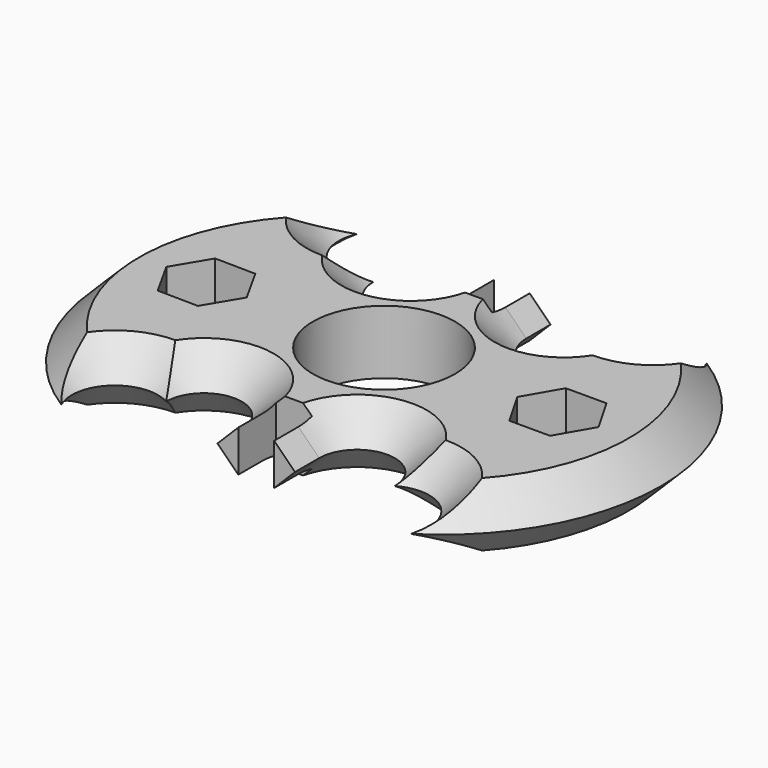
from build123d import *

# Parameters (mm, degrees)
F0_R         = 11.125
F1_DEPTH     = 10
F2_T1_DEPTH  = 17.5952575274
F2_T3_DEPTH  = 17.5952575274
F2_T6_ANGLE  = 359.64
F2_T8_ANGLE  = 359.64
F2_T10_ANGLE = 158.7108465942
F2_T12_ANGLE = 359.64
F2_T14_ANGLE = 359.64
F2_T16_ANGLE = 359.64
F2_T18_ANGLE = 359.64
F2_T20_ANGLE = 158.7108465942
F2_T22_ANGLE = 359.64
F2_T24_ANGLE = 359.64
F2_T26_ANGLE = 359.64
F2_T28_ANGLE = 158.7108465942
F2_T30_ANGLE = 359.64
F2_T32_ANGLE = 359.64
F2_T34_ANGLE = 359.64
F2_T36_ANGLE = 359.64
F2_T38_ANGLE = 359.64
F2_T40_ANGLE = 359.64
F2_T42_ANGLE = 158.7108465942
F2_T44_ANGLE = 359.64


# Not quite as in the source:
# - a fillet or chamfer that OpenCascade refuses, or shapes differently, is made with other operations: its cross-section is extruded or revolved along the edge and cut away or added


with BuildPart() as f1:
    # F0 (on Top) → F1 (new body)
    with BuildSketch(Plane.XY):
        with BuildLine():
            Line((-2.8125022072, -17.6151320338), (0, -17.6151320338))
            Line((0, -17.6151320338), (2.8125022072, -17.6151320338))
            Line((2.8125022072, -17.6151320338), (2.8125022072, -25.0164493918))
            Line((2.8125022072, -25.0164493918), (6.0690809041, -25.0164493918))
            Line((6.0690809041, -25.0164493918), (6.0690809041, -20.2796068043))
            ThreePointArc((6.0690809041, -20.2796068043), (11.9901318103, -14.3585558981), (17.9111827165, -20.2796068043))
            ThreePointArc((17.9111827165, -20.2796068043), (25.8046814323, -21.1516241303), (27.4031855301, -28.930603552))
            ThreePointArc((27.4031855301, -28.930603552), (43.3717109263, 0), (27.4031855301, 28.930603552))
            ThreePointArc((27.4031855301, 28.930603552), (25.8046814323, 21.1516241303), (17.9111827165, 20.2796068043))
            ThreePointArc((17.9111827165, 20.2796068043), (11.9901318103, 14.3585558981), (6.0690809041, 20.2796068043))
            Line((6.0690809041, 20.2796068043), (6.0690809041, 25.0164493918))
            Line((6.0690809041, 25.0164493918), (2.8125022072, 25.0164493918))
            Line((2.8125022072, 25.0164493918), (2.8125022072, 17.6151320338))
            Line((2.8125022072, 17.6151320338), (0, 17.6151320338))
            Line((0, 17.6151320338), (-2.8125022072, 17.6151320338))
            Line((-2.8125022072, 17.6151320338), (-2.8125022072, 25.0164493918))
            Line((-2.8125022072, 25.0164493918), (-6.0690809041, 25.0164493918))
            Line((-6.0690809041, 25.0164493918), (-6.0690809041, 20.2796068043))
            ThreePointArc((-6.0690809041, 20.2796068043), (-11.9901318103, 14.3585558981), (-17.9111827165, 20.2796068043))
            ThreePointArc((-17.9111827165, 20.2796068043), (-25.8046814323, 21.1516241303), (-27.4031855301, 28.930603552))
            ThreePointArc((-27.4031855301, 28.930603552), (-43.3717109263, 0), (-27.4031855301, -28.930603552))
            ThreePointArc((-27.4031855301, -28.930603552), (-25.8046814323, -21.1516241303), (-17.9111827165, -20.2796068043))
            ThreePointArc((-17.9111827165, -20.2796068043), (-11.9901318103, -14.3585558981), (-6.0690809041, -20.2796068043))
            Line((-6.0690809041, -20.2796068043), (-6.0690809041, -25.0164493918))
            Line((-6.0690809041, -25.0164493918), (-2.8125022072, -25.0164493918))
            Line((-2.8125022072, -25.0164493918), (-2.8125022072, -17.6151320338))
        make_face()
        Polygon((-30.9119913686, 5.5693711821), (-24.537748198, 5.4711418492), (-21.4356957103, -0.0982293328), (-24.7078863932, -5.5693711821), (-31.0821295639, -5.4711418492), (-34.1841820515, 0.0982293328), align=None, mode=Mode.SUBTRACT)
        Circle(F0_R, mode=Mode.SUBTRACT)
        Polygon((20.875, 0), (24.0625, 5.5209119491), (30.4375, 5.5209119491), (33.625, 0), (30.4375, -5.5209119491), (24.0625, -5.5209119491), align=None, mode=Mode.SUBTRACT)
    extrude(amount=F1_DEPTH)

    # F2: chamfer of 5 on 20 edges, made by hand

    # F2_s2 → F2_t1 (cut)
    with BuildSketch(Plane.XZ.offset(-37.8748643317)):
        Polygon((-6.0690809041, 5), (-1.0690809041, 0), (-6.0690809041, 0), align=None)
        Polygon((6.0690809041, 5), (1.0690809041, 0), (6.0690809041, 0), align=None)
        Polygon((1.0690809041, 10), (6.0690809041, 5), (6.0690809041, 10), align=None)
        Polygon((-1.0690809041, 10), (-6.0690809041, 5), (-6.0690809041, 10), align=None)
    extrude(amount=F2_T1_DEPTH, mode=Mode.SUBTRACT)

    # F2_s4 → F2_t3 (cut)
    with BuildSketch(Plane.XZ.offset(20.2796068043)):
        Polygon((-1.0690809041, 0), (-6.0690809041, 5), (-6.0690809041, 0), align=None)
        Polygon((6.0690809041, 5), (1.0690809041, 0), (6.0690809041, 0), align=None)
        Polygon((1.0690809041, 10), (6.0690809041, 5), (6.0690809041, 10), align=None)
        Polygon((-1.0690809041, 10), (-6.0690809041, 5), (-6.0690809041, 10), align=None)
    extrude(amount=F2_T3_DEPTH, mode=Mode.SUBTRACT)

    # F2_s5 → F2_t6 (revolve, cut)
    with BuildSketch(Plane(origin=(-24.5672156268, 22.5322183518, 0), x_dir=(0, 0, 1), z_dir=(-0.7369707586, 0.6759246267, 0))):
        Polygon((10, 16.6434047939), (5, 11.6434047939), (10, 11.6434047939), align=None)
    revolve(axis=Axis((-21.2587402157, 26.1394987159, 10), (0, 0, -1)), revolution_arc=F2_T6_ANGLE, mode=Mode.SUBTRACT)

    # F2_s7 → F2_t8 (revolve, cut)
    with BuildSketch(Plane.XZ.offset(-20.2796068043)):
        Polygon((-1.0690809041, 10), (-6.0690809041, 5), (-6.0690809041, 10), align=None)
    revolve(axis=Axis((-11.9901318103, 20.2796068043, 10), (0, 0, -1)), revolution_arc=F2_T8_ANGLE, mode=Mode.SUBTRACT)

    # F2_s9 → F2_t10 (revolve, cut)
    with BuildSketch(Plane(origin=(-8.8670439331, -1.6665634724, 0), x_dir=(0, 0, 1), z_dir=(0.9827919356, 0.1847160286, 0))):
        Polygon((10, -30.8871798498), (5, -35.8871798498), (10, -35.8871798498), align=None)
    revolve(axis=Axis((-9.1802750199, 0, 10), (0, 0, 1)), revolution_arc=F2_T10_ANGLE, mode=Mode.SUBTRACT)

    # F2_s11 → F2_t12 (revolve, cut)
    with BuildSketch(Plane(origin=(-24.6850209159, -22.3563277123, 0), x_dir=(0, 0, 1), z_dir=(0.7412031432, 0.6712807911, 0))):
        Polygon((10, 16.8527592984), (5, 11.8527592984), (10, 11.8527592984), align=None)
    revolve(axis=Axis((-21.2587402157, -26.1394987159, 10), (0, 0, -1)), revolution_arc=F2_T12_ANGLE, mode=Mode.SUBTRACT)

    # F2_s13 → F2_t14 (revolve, cut)
    with BuildSketch(Plane(origin=(-0.1278905192, -20.3541404453, 0), x_dir=(0, 0, 1), z_dir=(0.006283144, 0.9999802609, 0))):
        Polygon((5, -5.9414245401), (10, -0.9414245401), (10, -5.9414245401), align=None)
    revolve(axis=Axis((-11.9901318103, -20.2796068043, 10), (0, 0, -1)), revolution_arc=F2_T14_ANGLE, mode=Mode.SUBTRACT)

    # F2_s15 → F2_t16 (revolve, cut)
    with BuildSketch(Plane.XZ.offset(20.2796068043)):
        Polygon((1.0690809041, 10), (6.0690809041, 5), (6.0690809041, 10), align=None)
    revolve(axis=Axis((11.9901318103, -20.2796068043, 10), (0, 0, -1)), revolution_arc=F2_T16_ANGLE, mode=Mode.SUBTRACT)

    # F2_s17 → F2_t18 (revolve, cut)
    with BuildSketch(Plane(origin=(24.5672156268, -22.5322183518, 0), x_dir=(0, 0, 1), z_dir=(0.7369707586, -0.6759246267, 0))):
        Polygon((10, 16.6434047939), (5, 11.6434047939), (10, 11.6434047939), align=None)
    revolve(axis=Axis((21.2587402157, -26.1394987159, 10), (0, 0, -1)), revolution_arc=F2_T18_ANGLE, mode=Mode.SUBTRACT)

    # F2_s19 → F2_t20 (revolve, cut)
    with BuildSketch(Plane(origin=(8.8670439331, 1.6665634724, 0), x_dir=(0, 0, 1), z_dir=(-0.9827919356, -0.1847160286, 0))):
        Polygon((10, -30.8871798498), (5, -35.8871798498), (10, -35.8871798498), align=None)
    revolve(axis=Axis((9.1802750199, 0, 10), (0, 0, 1)), revolution_arc=F2_T20_ANGLE, mode=Mode.SUBTRACT)

    # F2_s21 → F2_t22 (revolve, cut)
    with BuildSketch(Plane(origin=(24.6850209159, 22.3563277123, 0), x_dir=(0, 0, 1), z_dir=(-0.7412031432, -0.6712807911, 0))):
        Polygon((10, 16.8527592984), (5, 11.8527592984), (10, 11.8527592984), align=None)
    revolve(axis=Axis((21.2587402157, 26.1394987159, 10), (0, 0, -1)), revolution_arc=F2_T22_ANGLE, mode=Mode.SUBTRACT)

    # F2_s23 → F2_t24 (revolve, cut)
    with BuildSketch(Plane(origin=(0.1278905192, 20.3541404453, 0), x_dir=(0, 0, 1), z_dir=(-0.006283144, -0.9999802609, 0))):
        Polygon((10, -0.9414245401), (5, -5.9414245401), (10, -5.9414245401), align=None)
    revolve(axis=Axis((11.9901318103, 20.2796068043, 10), (0, 0, -1)), revolution_arc=F2_T24_ANGLE, mode=Mode.SUBTRACT)

    # F2_s25 → F2_t26 (revolve, cut)
    with BuildSketch(Plane(origin=(24.6850209159, 22.3563277123, 0), x_dir=(0, 0, 1), z_dir=(-0.7412031432, -0.6712807911, 0))):
        Polygon((5, 11.8527592984), (0, 16.8527592984), (0, 11.8527592984), align=None)
    revolve(axis=Axis((21.2587402157, 26.1394987159, 0), (0, 0, -1)), revolution_arc=F2_T26_ANGLE, mode=Mode.SUBTRACT)

    # F2_s27 → F2_t28 (revolve, cut)
    with BuildSketch(Plane(origin=(8.8670439331, 1.6665634724, 0), x_dir=(0, 0, 1), z_dir=(-0.9827919356, -0.1847160286, 0))):
        Polygon((5, -35.8871798498), (0, -30.8871798498), (0, -35.8871798498), align=None)
    revolve(axis=Axis((9.1802750199, 0, 0), (0, 0, 1)), revolution_arc=F2_T28_ANGLE, mode=Mode.SUBTRACT)

    # F2_s29 → F2_t30 (revolve, cut)
    with BuildSketch(Plane(origin=(24.5672156268, -22.5322183518, 0), x_dir=(0, 0, 1), z_dir=(0.7369707586, -0.6759246267, 0))):
        Polygon((5, 11.6434047939), (0, 16.6434047939), (0, 11.6434047939), align=None)
    revolve(axis=Axis((21.2587402157, -26.1394987159, 0), (0, 0, -1)), revolution_arc=F2_T30_ANGLE, mode=Mode.SUBTRACT)

    # F2_s31 → F2_t32 (revolve, cut)
    with BuildSketch(Plane.XZ.offset(20.2796068043)):
        Polygon((6.0690809041, 5), (1.0690809041, 0), (6.0690809041, 0), align=None)
    revolve(axis=Axis((11.9901318103, -20.2796068043, 0), (0, 0, -1)), revolution_arc=F2_T32_ANGLE, mode=Mode.SUBTRACT)

    # F2_s33 → F2_t34 (revolve, cut)
    with BuildSketch(Plane(origin=(-0.1278905192, -20.3541404453, 0), x_dir=(0, 0, 1), z_dir=(0.006283144, 0.9999802609, 0))):
        Polygon((5, -5.9414245401), (0, -0.9414245401), (0, -5.9414245401), align=None)
    revolve(axis=Axis((-11.9901318103, -20.2796068043, 0), (0, 0, -1)), revolution_arc=F2_T34_ANGLE, mode=Mode.SUBTRACT)

    # F2_s35 → F2_t36 (revolve, cut)
    with BuildSketch(Plane(origin=(0.1278905192, 20.3541404453, 0), x_dir=(0, 0, 1), z_dir=(-0.006283144, -0.9999802609, 0))):
        Polygon((5, -5.9414245401), (0, -0.9414245401), (0, -5.9414245401), align=None)
    revolve(axis=Axis((11.9901318103, 20.2796068043, 0), (0, 0, -1)), revolution_arc=F2_T36_ANGLE, mode=Mode.SUBTRACT)

    # F2_s37 → F2_t38 (revolve, cut)
    with BuildSketch(Plane.XZ.offset(-20.2796068043)):
        Polygon((-6.0690809041, 5), (-1.0690809041, 0), (-6.0690809041, 0), align=None)
    revolve(axis=Axis((-11.9901318103, 20.2796068043, 0), (0, 0, -1)), revolution_arc=F2_T38_ANGLE, mode=Mode.SUBTRACT)

    # F2_s39 → F2_t40 (revolve, cut)
    with BuildSketch(Plane(origin=(-24.5672156268, 22.5322183518, 0), x_dir=(0, 0, 1), z_dir=(-0.7369707586, 0.6759246267, 0))):
        Polygon((5, 11.6434047939), (0, 16.6434047939), (0, 11.6434047939), align=None)
    revolve(axis=Axis((-21.2587402157, 26.1394987159, 0), (0, 0, -1)), revolution_arc=F2_T40_ANGLE, mode=Mode.SUBTRACT)

    # F2_s41 → F2_t42 (revolve, cut)
    with BuildSketch(Plane(origin=(-8.8670439331, -1.6665634724, 0), x_dir=(0, 0, 1), z_dir=(0.9827919356, 0.1847160286, 0))):
        Polygon((5, -35.8871798498), (0, -30.8871798498), (0, -35.8871798498), align=None)
    revolve(axis=Axis((-9.1802750199, 0, 0), (0, 0, 1)), revolution_arc=F2_T42_ANGLE, mode=Mode.SUBTRACT)

    # F2_s43 → F2_t44 (revolve, cut)
    with BuildSketch(Plane(origin=(-24.6850209159, -22.3563277123, 0), x_dir=(0, 0, 1), z_dir=(0.7412031432, 0.6712807911, 0))):
        Polygon((0, 16.8527592984), (5, 11.8527592984), (0, 11.8527592984), align=None)
    revolve(axis=Axis((-21.2587402157, -26.1394987159, 0), (0, 0, -1)), revolution_arc=F2_T44_ANGLE, mode=Mode.SUBTRACT)


solid = f1.part
